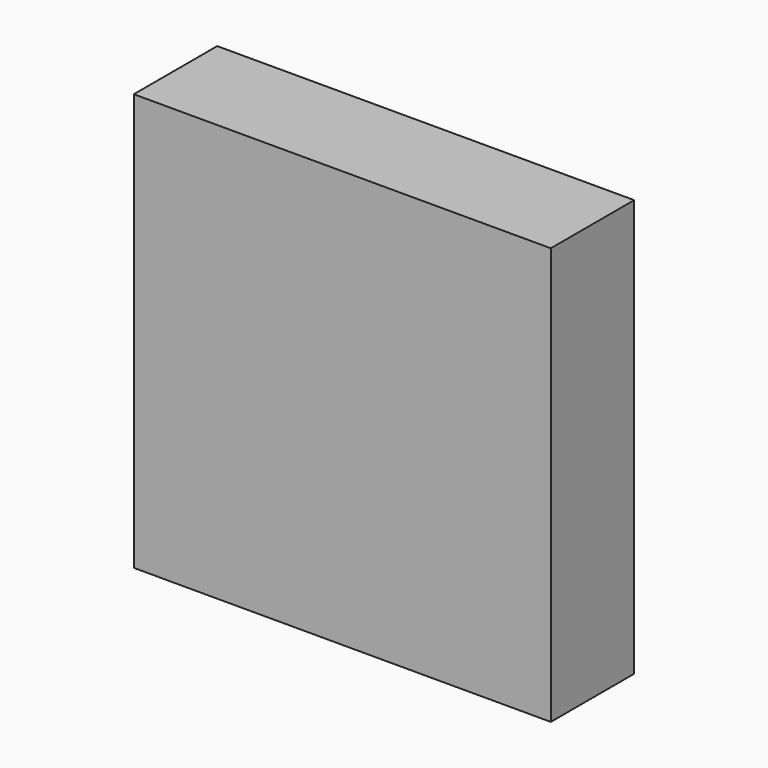
from build123d import *

# Parameters (mm, degrees)
F0_W     = 100
F0_H     = 100
F1_DEPTH = 25


# Not quite as in the source:
# - the program builds the solid bodies; features that only make, move or delete a surface that nothing else refers to are left out


with BuildPart() as f1:
    # F0 (on Front) → F1 (new body)
    with BuildSketch(Plane.XZ):
        with Locations((50, -50)):
            Rectangle(F0_W, F0_H)
    extrude(amount=F1_DEPTH)


solid = f1.part
